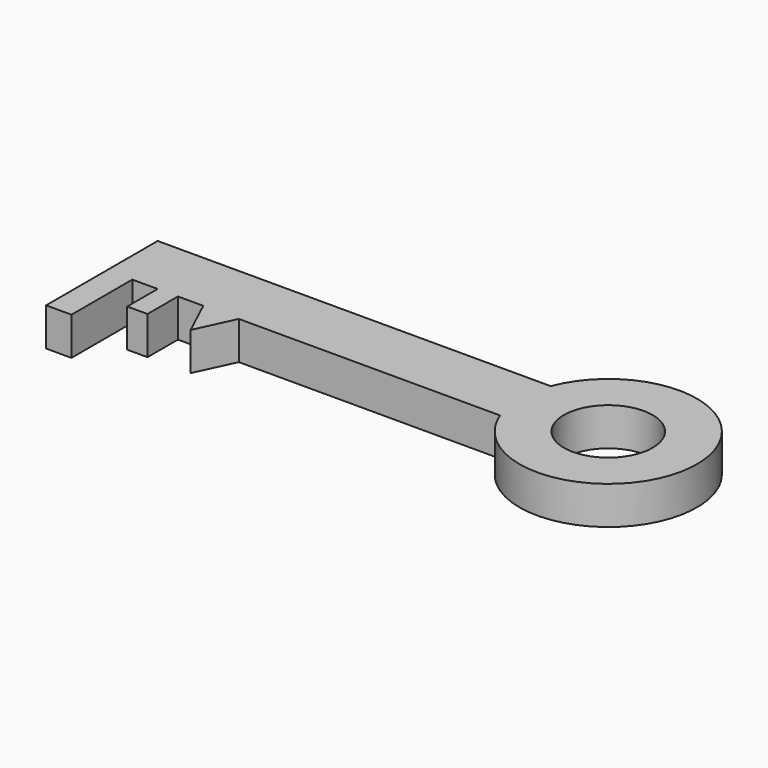
from build123d import *

# Parameters (mm, degrees)
F0_W     = 8
F0_H     = 15
F0_W_2   = 10
F0_H_2   = 30
F0_R     = 17.5
F1_DEPTH = 15


# Not quite as in the source:
# - a feature of the source that left no trace in its solid (it failed there, or was rolled back) is left out


with BuildPart() as f1:
    # F0 (on Top) → F1 (new body)
    with BuildSketch(Plane.XY):
        Polygon((76.7292545206, 57.9236412775), (-78.2707454794, 57.9236412775), (-78.2707454794, 32.9236412775), (-68.2707454794, 32.9236412775), (-58.2707454794, 32.9236412775), (-50.2707454794, 32.9236412775), (-40.2707454794, 32.9236412775), (-26.2707454794, 32.9236412775), (76.7292545206, 32.9236412775), align=None)
        Polygon((-33.2707454794, 17.9236412775), (-26.2707454794, 32.9236412775), (-40.2707454794, 32.9236412775), align=None)
        with Locations((-54.2707454794, 25.4236412775)):
            Rectangle(F0_W, F0_H)
        with Locations((-73.2707454794, 17.9236412775)):
            Rectangle(F0_W_2, F0_H_2)
        with BuildLine():
            ThreePointArc((76.7292545206, 32.9236412775), (144.4209965971, 45.4236412775), (76.7292545206, 57.9236412775))
            Line((76.7292545206, 57.9236412775), (76.7292545206, 32.9236412775))
        make_face()
        with Locations((109.4209965971, 45.4236412775)):
            Circle(F0_R, mode=Mode.SUBTRACT)
    extrude(amount=F1_DEPTH)


solid = f1.part
